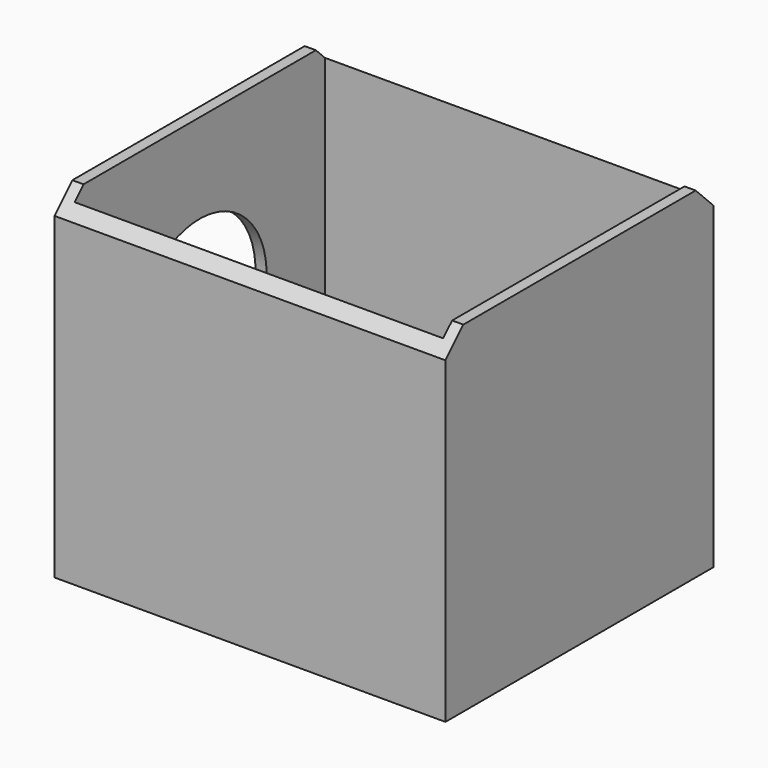
from build123d import *

# Parameters (mm, degrees)
F0_W        = 35
F0_H        = 30
F1_DEPTH    = 30.5
F2_T        = -1
F4_D        = 15
F4_DEPTH    = 12
F4_TIP      = 4.5064546427
F5_T1_DEPTH = 45.2867319519
F6_T1_DEPTH = 45.2867319519


# Not quite as in the source:
# - a fillet or chamfer that OpenCascade refuses, or shapes differently, is made with other operations: its cross-section is extruded or revolved along the edge and cut away or added


with BuildPart() as f1:
    # F0 (on Top) → F1 (new body)
    with BuildSketch(Plane.XY):
        with Locations((17.5, 15)):
            Rectangle(F0_W, F0_H)
    extrude(amount=F1_DEPTH)

    # F2
    f2_openings = [f1.faces().sort_by_distance(p)[0] for p in [
        (17.5, 15, 30.5),
    ]]
    offset(amount=F2_T, openings=f2_openings)

    # F4
    with Locations(Plane(origin=(0, 0, 0), x_dir=(0, 1, 0), z_dir=(-1, 0, 0))):
        with Locations((15, -15)):
            Hole(F4_D / 2, depth=F4_DEPTH)
            with Locations((0, 0, -(F4_DEPTH + F4_TIP / 2))):  # 118° drill point
                Cone(0, F4_D / 2, F4_TIP, mode=Mode.SUBTRACT)

    # F5: chamfer of 2 on 1 edges, made by hand

    # F5_s2 → F5_t1 (cut)
    with BuildSketch(Plane.YZ.offset(-5.1433659759)):
        Polygon((2, 30.5), (0, 28.5), (0, 30.5), align=None)
    extrude(amount=F5_T1_DEPTH, mode=Mode.SUBTRACT)

    # F6: chamfer of 2 on 1 edges, made by hand

    # F6_s2 → F6_t1 (cut)
    with BuildSketch(Plane.YZ.offset(-5.1433659759)):
        Polygon((28, 30.5), (30, 28.5), (30, 30.5), align=None)
    extrude(amount=F6_T1_DEPTH, mode=Mode.SUBTRACT)


solid = f1.part
